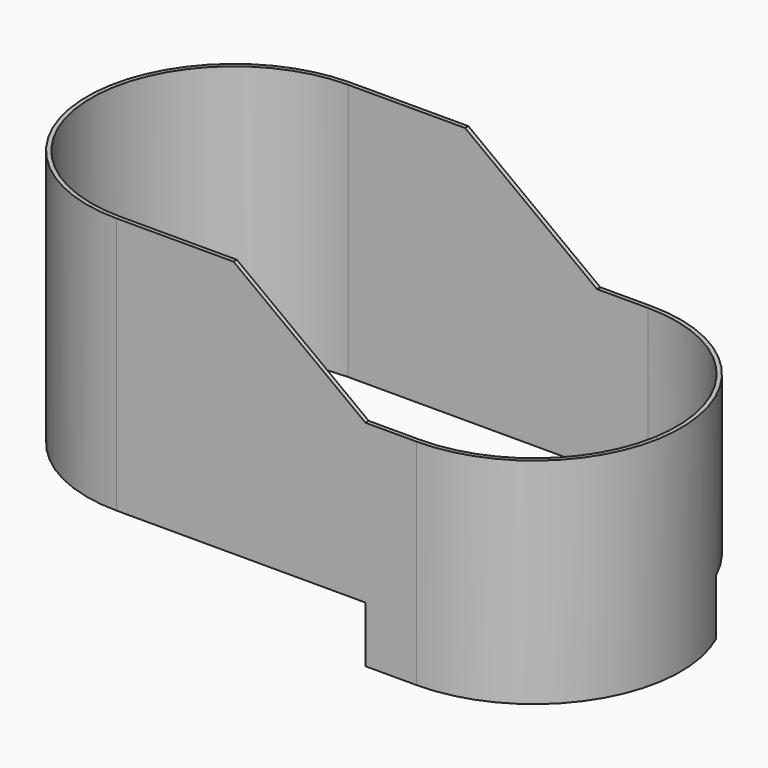
from build123d import *

# Parameters (mm, degrees)
F0_W     = 231.14
F0_H     = 226.06
F1_DEPTH = 241.3
F2_W     = 113.03
F2_H     = 76.2
F2_W_2   = 39.37
F2_W_3   = 150.0068409762
F2_H_2   = 43.18
F2_W_4   = 191.77
F3_DEPTH = 226.061
F6_DEPTH = 241.301
F4_W     = 102.87
F4_H     = 43.18
F4_W_2   = 39.37
F7_DEPTH = 114.046


# Not quite as in the source:
# - a feature names something its author has since deleted; it is built from what else it names


with BuildPart() as f1:
    # F0 (on Top) → F1 (new body)
    with BuildSketch(Plane.XY):
        with BuildLine():
            Line((-173.0334059873, -173.7446556775), (-173.0334059873, 52.3153443225))
            ThreePointArc((-173.0334059873, 52.3153443225), (-286.0634059873, -60.7146556775), (-173.0334059873, -173.7446556775))
        make_face()
        with Locations((-57.4634059873, -60.7146556775)):
            Rectangle(F0_W, F0_H)
        with BuildLine():
            ThreePointArc((58.1065940127, -173.7446556775), (171.1365940127, -60.7146556775), (58.1065940127, 52.3153443225))
            Line((58.1065940127, 52.3153443225), (58.1065940127, -173.7446556775))
        make_face()
    extrude(amount=F1_DEPTH)

    # F2 (on face) → F3 (cut, through all)
    with BuildSketch(Plane.XZ.offset(173.7446556775)):
        Polygon((18.7365940127, 241.3), (-82.8634059873, 241.3), (18.7365940127, 165.1), align=None)
        with Locations((114.6215940127, 203.2)):
            Rectangle(F2_W, F2_H)
        with Locations((38.4215940127, 203.2)):
            Rectangle(F2_W_2, F2_H)
        with Locations((-248.0368264754, 21.59)):
            Rectangle(F2_W_3, F2_H_2)
        with Locations((-77.1484059873, 21.59)):
            Rectangle(F2_W_4, F2_H_2)
    extrude(amount=-F3_DEPTH, mode=Mode.SUBTRACT)

    # F5 (on face) → F6 (cut, through all)
    with BuildSketch(Plane(origin=(0, 0, 0), x_dir=(1, 0, 0), z_dir=(0, 0, -1))):
        with BuildLine():
            ThreePointArc((-173.0334059873, 170.5696556775), (-282.8884059873, 60.7146556775), (-173.0334059873, -49.1403443225))
            Line((-173.0334059873, -49.1403443225), (3.4965941633, -49.1403443225))
            Line((3.4965941633, -49.1403443225), (18.7365940127, -49.1403443225))
            Line((18.7365940127, -49.1403443225), (18.7365940127, 170.5696556775))
            Line((18.7365940127, 170.5696556775), (3.4965941633, 170.5696556775))
            Line((3.4965941633, 170.5696556775), (-173.0334059873, 170.5696556775))
        make_face()
        with BuildLine():
            Line((18.7365940127, 170.5696556775), (18.7365940127, -49.1403443225))
            Line((18.7365940127, -49.1403443225), (21.9115940127, -49.1403443225))
            Line((21.9115940127, -49.1403443225), (58.1065940127, -49.1403443225))
            ThreePointArc((58.1065940127, -49.1403443225), (167.9615940127, 60.7146556775), (58.1065940127, 170.5696556775))
            Line((58.1065940127, 170.5696556775), (21.9115940127, 170.5696556775))
            Line((21.9115940127, 170.5696556775), (18.7365940127, 170.5696556775))
        make_face()
    extrude(amount=-F6_DEPTH, mode=Mode.SUBTRACT)

    # F4 (on face) → F7 (cut)
    with BuildSketch(Plane(origin=(0, 52.3153443225, 0), x_dir=(-1, 0, 0), z_dir=(0, 1, 0))):
        with Locations((-109.5415940127, 21.59)):
            Rectangle(F4_W, F4_H)
        with Locations((-38.4215940127, 21.59)):
            Rectangle(F4_W_2, F4_H)
    extrude(amount=-F7_DEPTH, mode=Mode.SUBTRACT)


solid = f1.part
